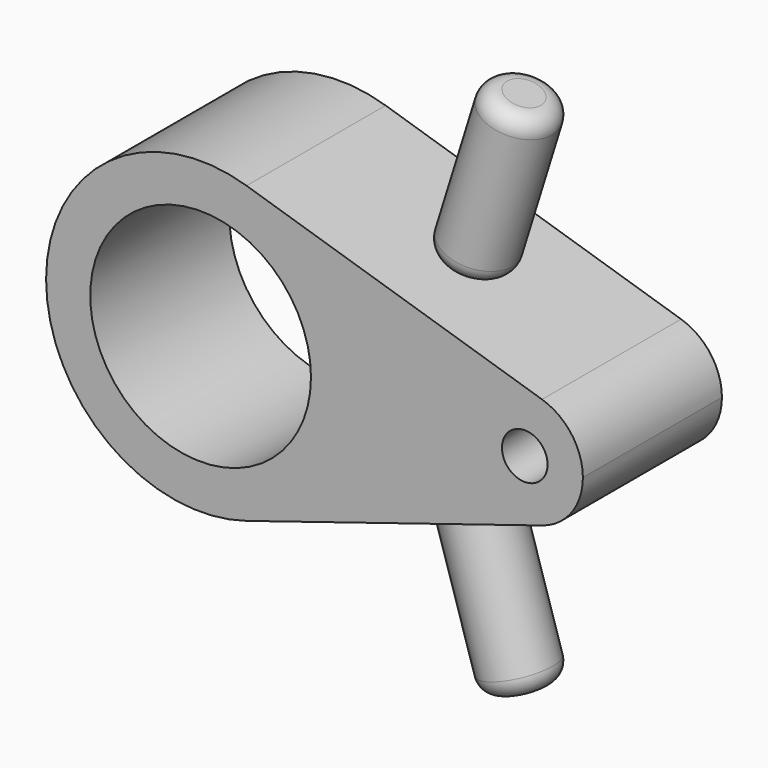
from build123d import *

# Parameters (mm, degrees)
F0_R     = 31.75
F1_DEPTH = 50
F2_R     = 10.16
F3_DEPTH = 49.022
F4_R     = 5.08
F5_R     = 6.5584934957
F6_DEPTH = 50.001


with BuildPart() as f1:
    # F0 (on Front) → F1 (new body)
    with BuildSketch(Plane.XZ):
        with BuildLine():
            ThreePointArc((13.2197323108, -42.4386754934), (35.8009748556, -26.3456390963), (44.45, 0))
            ThreePointArc((44.45, 0), (35.8009748556, 26.3456390963), (13.2197323108, 42.4386754934))
            ThreePointArc((13.2197323108, 42.4386754934), (-44.45, 0), (13.2197323108, -42.4386754934))
        make_face()
        Circle(F0_R, mode=Mode.SUBTRACT)
        with BuildLine():
            ThreePointArc((13.2197323108, 42.4386754934), (35.8009748556, 26.3456390963), (44.45, 0))
            ThreePointArc((44.45, 0), (35.8009748556, -26.3456390963), (13.2197323108, -42.4386754934))
            Line((13.2197323108, -42.4386754934), (98.2165525677, -15.9619959551))
            ThreePointArc((98.2165525677, -15.9619959551), (76.5258654015, 0), (98.2165525677, 15.9619959551))
            Line((98.2165525677, 15.9619959551), (13.2197323108, 42.4386754934))
        make_face()
        with BuildLine():
            ThreePointArc((109.9628523929, 0), (106.7097889369, 9.9090977699), (98.2165525677, 15.9619959551))
            ThreePointArc((98.2165525677, 15.9619959551), (76.5258654015, 0), (98.2165525677, -15.9619959551))
            ThreePointArc((98.2165525677, -15.9619959551), (106.7097889369, -9.9090977699), (109.9628523929, 0))
        make_face()
    extrude(amount=F1_DEPTH)

    # F5 (on face) → F6 (cut, through all)
    with BuildSketch(Plane.XZ.offset(50)):
        with Locations((93.2443588972, 0)):
            Circle(F5_R)
    extrude(amount=-F6_DEPTH, mode=Mode.SUBTRACT)



with BuildPart() as f3:
    # F2 (on face) → F3 (new body)
    with BuildSketch(Plane(origin=(13.2197323108, 0, 42.4386754934), x_dir=(0.9547508547, 0, -0.2974068011), z_dir=(0.2974068011, 0, 0.9547508547))):
        with Locations((47.3798899133, -25)):
            Circle(F2_R)
    extrude(amount=F3_DEPTH)

    # F4
    f4_edges = [f3.edges().sort_by_distance(p)[0] for p in [
        (63.33493, -25, 78.173023),
        (48.755454, -25, 31.369227),
    ]]
    fillet(f4_edges, radius=F4_R)


with BuildPart() as f1_1:
    add(f1.part)

    add(f3.part)  # F7 merges F3
    # F7: F3 across plane
    add(f3.part.mirror(Plane.XY))


solid = f1_1.part
